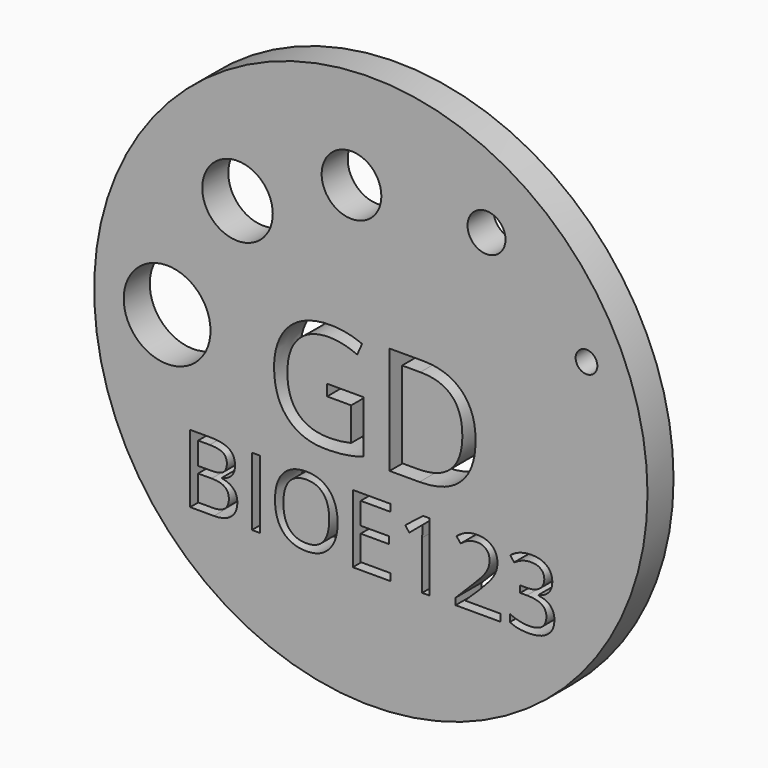
from build123d import *

# Parameters (mm, degrees)
F0_R         = 25.5
F1_DEPTH     = 3
F2_R         = 4
F2_R_2       = 3.25
F2_R_3       = 2.75
F2_R_4       = 1.75
F2_R_5       = 1
F3_DEPTH     = 3
F4_TEXT_SIZE = 8.7874151661
F5_DEPTH     = 3
F6_TEXT_SIZE = 13.9109696546
F7_DEPTH     = 3


# Not quite as in the source:
# - Text() gives the source's letters only with a copy of the font that has no kerning and outlines rounded to 1/6400 em; it was checked with that copy


with BuildPart() as f1:
    # F0 (on Front) → F1 (new body)
    with BuildSketch(Plane.XZ):
        Circle(F0_R)
    extrude(amount=F1_DEPTH)

    # F2 (on Front) → F3 (cut)
    with BuildSketch(Plane.XZ):
        with Locations((-18.7770126888, 0.1230475614)):
            Circle(F2_R)
        with Locations((-12.2891567254, 11.4695964454)):
            Circle(F2_R_2)
        with Locations((-1.7820451399, 16.1669889818)):
            Circle(F2_R_3)
        with Locations((10.6604207564, 16.3626791907)):
            Circle(F2_R_4)
        with Locations((19.8733744793, 8.8626512288)):
            Circle(F2_R_5)
    extrude(amount=F3_DEPTH, mode=Mode.SUBTRACT)

    # F4 (on Front) → F5 (cut)
    with BuildSketch(Plane.XZ):
        with Locations((-17.515212566, -14.8005186402)):
            Text('BIOE123', F4_TEXT_SIZE, font='Open Sans', text_align=(TextAlign.LEFT, TextAlign.BOTTOM))
    extrude(amount=F5_DEPTH, mode=Mode.SUBTRACT)

    # F6 (on Front) → F7 (cut)
    with BuildSketch(Plane.XZ):
        with Locations((-9.7655025311, -5.884340062)):
            Text('GD', F6_TEXT_SIZE, font='Open Sans', text_align=(TextAlign.LEFT, TextAlign.BOTTOM))
    extrude(amount=F7_DEPTH, mode=Mode.SUBTRACT)


solid = f1.part
